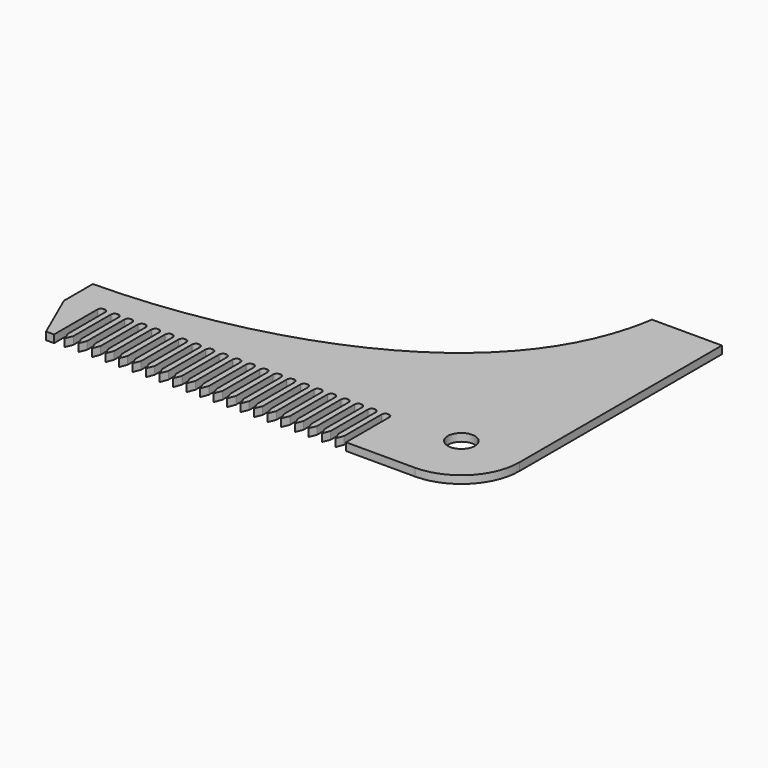
from build123d import *

# Parameters (mm, degrees)
F1_DEPTH = 2
F2_R     = 3.5
F3_DEPTH = 25


# Not quite as in the source:
# - a feature names something its author has since deleted; it is built from what else it names


with BuildPart() as f1:
    # F0 (on Top) → F1 (new body)
    with BuildSketch(Plane.XY):
        with BuildLine():
            ThreePointArc((-15.75, -19.0369902551), (-15.0428932188, -19.3298834739), (-14.75, -20.0369902551))
            Line((-14.75, -20.0369902551), (-14.75, -34))
            Line((-14.75, -34), (3.0843058825, -34))
            ThreePointArc((3.0843058825, -34), (13.6909076003, -29.6066017178), (18.0843058825, -19))
            Line((18.0843058825, -19), (18.0843058825, 46.4938916266))
            Line((18.0843058825, 46.4938916266), (0, 46.4938916266))
            add(Edge.make_bspline(
                [(-97.9156941175, -11.8882479146), (-60.4824349284, -11.5448236465), (-6.9082397968, 2.1921501029), (0, 46.4938916266)],
                knots=[0, 0, 0, 0, 113.9998130346, 113.9998130346, 113.9998130346, 113.9998130346], degree=3))
            Line((-97.9156941175, -11.8882479146), (-97.9156941175, -21.2501913908))
            Line((-97.9156941175, -21.2501913908), (-92.3223271966, -34))
            Line((-92.3223271966, -34), (-90.25, -34))
            Line((-90.25, -34), (-90.25, -32.1302767694))
            Line((-90.25, -32.1302767694), (-90.25, -20.0369902551))
            ThreePointArc((-90.25, -20.0369902551), (-89.9571067812, -19.3298834739), (-89.25, -19.0369902551))
            ThreePointArc((-89.25, -19.0369902551), (-88.5428932188, -19.3298834739), (-88.25, -20.0369902551))
            Line((-88.25, -20.0369902551), (-88.25, -32.1302767694))
            Line((-88.25, -32.1302767694), (-87.5, -34))
            Line((-87.5, -34), (-86.75, -32.1302767694))
            Line((-86.75, -32.1302767694), (-86.75, -20.0369902551))
            ThreePointArc((-86.75, -20.0369902551), (-86.4571067812, -19.3298834739), (-85.75, -19.0369902551))
            ThreePointArc((-85.75, -19.0369902551), (-85.0428932188, -19.3298834739), (-84.75, -20.0369902551))
            Line((-84.75, -20.0369902551), (-84.75, -32.1025866866))
            Line((-84.75, -32.1025866866), (-84, -34))
            Line((-84, -34), (-83.25, -32.1025866866))
            Line((-83.25, -32.1025866866), (-83.25, -20.0369902551))
            ThreePointArc((-83.25, -20.0369902551), (-82.9571067812, -19.3298834739), (-82.25, -19.0369902551))
            ThreePointArc((-82.25, -19.0369902551), (-81.5428932188, -19.3298834739), (-81.25, -20.0369902551))
            Line((-81.25, -20.0369902551), (-81.25, -32.0932865143))
            Line((-81.25, -32.0932865143), (-80.5, -34))
            Line((-80.5, -34), (-79.75, -32.0932865143))
            Line((-79.75, -32.0932865143), (-79.75, -20.0369902551))
            ThreePointArc((-79.75, -20.0369902551), (-79.4571067812, -19.3298834739), (-78.75, -19.0369902551))
            ThreePointArc((-78.75, -19.0369902551), (-78.0428932188, -19.3298834739), (-77.75, -20.0369902551))
            Line((-77.75, -20.0369902551), (-77.75, -32.0655964315))
            Line((-77.75, -32.0655964315), (-77, -34))
            Line((-77, -34), (-76.25, -32.0655964315))
            Line((-76.25, -32.0655964315), (-76.25, -20.0369902551))
            ThreePointArc((-76.25, -20.0369902551), (-75.9571067812, -19.3298834739), (-75.25, -19.0369902551))
            ThreePointArc((-75.25, -19.0369902551), (-74.5428932188, -19.3298834739), (-74.25, -20.0369902551))
            Line((-74.25, -20.0369902551), (-74.25, -32.0655964315))
            Line((-74.25, -32.0655964315), (-73.5, -34))
            Line((-73.5, -34), (-72.75, -32.0655964315))
            Line((-72.75, -32.0655964315), (-72.75, -20.0369902551))
            ThreePointArc((-72.75, -20.0369902551), (-72.4571067812, -19.3298834739), (-71.75, -19.0369902551))
            ThreePointArc((-71.75, -19.0369902551), (-71.0428932188, -19.3298834739), (-70.75, -20.0369902551))
            Line((-70.75, -20.0369902551), (-70.75, -32.0932865143))
            Line((-70.75, -32.0932865143), (-70, -34))
            Line((-70, -34), (-69.25, -32.0932865143))
            Line((-69.25, -32.0932865143), (-69.25, -20.0369902551))
            ThreePointArc((-69.25, -20.0369902551), (-68.9571067812, -19.3298834739), (-68.25, -19.0369902551))
            ThreePointArc((-68.25, -19.0369902551), (-67.5428932188, -19.3298834739), (-67.25, -20.0369902551))
            Line((-67.25, -20.0369902551), (-67.25, -32.0932865143))
            Line((-67.25, -32.0932865143), (-66.5, -34))
            Line((-66.5, -34), (-65.75, -32.0932865143))
            Line((-65.75, -32.0932865143), (-65.75, -20.0369902551))
            ThreePointArc((-65.75, -20.0369902551), (-65.4571067812, -19.3298834739), (-64.75, -19.0369902551))
            ThreePointArc((-64.75, -19.0369902551), (-64.0428932188, -19.3298834739), (-63.75, -20.0369902551))
            Line((-63.75, -20.0369902551), (-63.75, -32.0655964315))
            Line((-63.75, -32.0655964315), (-63, -34))
            Line((-63, -34), (-62.25, -32.0655964315))
            Line((-62.25, -32.0655964315), (-62.25, -20.0369902551))
            ThreePointArc((-62.25, -20.0369902551), (-61.9571067812, -19.3298834739), (-61.25, -19.0369902551))
            ThreePointArc((-61.25, -19.0369902551), (-60.5428932188, -19.3298834739), (-60.25, -20.0369902551))
            Line((-60.25, -20.0369902551), (-60.25, -32.0655964315))
            Line((-60.25, -32.0655964315), (-59.5, -34))
            Line((-59.5, -34), (-58.75, -32.0655964315))
            Line((-58.75, -32.0655964315), (-58.75, -20.0369902551))
            ThreePointArc((-58.75, -20.0369902551), (-58.4571067812, -19.3298834739), (-57.75, -19.0369902551))
            ThreePointArc((-57.75, -19.0369902551), (-57.0428932188, -19.3298834739), (-56.75, -20.0369902551))
            Line((-56.75, -20.0369902551), (-56.75, -32.0932865143))
            Line((-56.75, -32.0932865143), (-56, -34))
            Line((-56, -34), (-55.25, -32.0932865143))
            Line((-55.25, -32.0932865143), (-55.25, -20.0369902551))
            ThreePointArc((-55.25, -20.0369902551), (-54.9571067812, -19.3298834739), (-54.25, -19.0369902551))
            ThreePointArc((-54.25, -19.0369902551), (-53.5428932188, -19.3298834739), (-53.25, -20.0369902551))
            Line((-53.25, -20.0369902551), (-53.25, -32.0932865143))
            Line((-53.25, -32.0932865143), (-52.5, -34))
            Line((-52.5, -34), (-51.75, -32.0932865143))
            Line((-51.75, -32.0932865143), (-51.75, -20.0369902551))
            ThreePointArc((-51.75, -20.0369902551), (-51.4571067812, -19.3298834739), (-50.75, -19.0369902551))
            ThreePointArc((-50.75, -19.0369902551), (-50.0428932188, -19.3298834739), (-49.75, -20.0369902551))
            Line((-49.75, -20.0369902551), (-49.75, -32.0655964315))
            Line((-49.75, -32.0655964315), (-49, -34))
            Line((-49, -34), (-48.25, -32.0655964315))
            Line((-48.25, -32.0655964315), (-48.25, -20.0369902551))
            ThreePointArc((-48.25, -20.0369902551), (-47.9571067812, -19.3298834739), (-47.25, -19.0369902551))
            ThreePointArc((-47.25, -19.0369902551), (-46.5428932188, -19.3298834739), (-46.25, -20.0369902551))
            Line((-46.25, -20.0369902551), (-46.25, -32.0655964315))
            Line((-46.25, -32.0655964315), (-45.5, -34))
            Line((-45.5, -34), (-44.75, -32.0655964315))
            Line((-44.75, -32.0655964315), (-44.75, -20.0369902551))
            ThreePointArc((-44.75, -20.0369902551), (-44.4571067812, -19.3298834739), (-43.75, -19.0369902551))
            ThreePointArc((-43.75, -19.0369902551), (-43.0428932188, -19.3298834739), (-42.75, -20.0369902551))
            Line((-42.75, -20.0369902551), (-42.75, -32.176785171))
            Line((-42.75, -32.176785171), (-42, -34))
            Line((-42, -34), (-41.25, -32.176785171))
            Line((-41.25, -32.176785171), (-41.25, -20.0369902551))
            ThreePointArc((-41.25, -20.0369902551), (-40.9571067812, -19.3298834739), (-40.25, -19.0369902551))
            ThreePointArc((-40.25, -19.0369902551), (-39.5428932188, -19.3298834739), (-39.25, -20.0369902551))
            Line((-39.25, -20.0369902551), (-39.25, -32.176785171))
            Line((-39.25, -32.176785171), (-38.5, -34))
            Line((-38.5, -34), (-37.75, -32.176785171))
            Line((-37.75, -32.176785171), (-37.75, -20.0369902551))
            ThreePointArc((-37.75, -20.0369902551), (-37.4571067812, -19.3298834739), (-36.75, -19.0369902551))
            ThreePointArc((-36.75, -19.0369902551), (-36.0428932188, -19.3298834739), (-35.75, -20.0369902551))
            Line((-35.75, -20.0369902551), (-35.75, -32.1490950882))
            Line((-35.75, -32.1490950882), (-35, -34))
            Line((-35, -34), (-34.25, -32.1490950882))
            Line((-34.25, -32.1490950882), (-34.25, -20.0369902551))
            ThreePointArc((-34.25, -20.0369902551), (-33.9571067812, -19.3298834739), (-33.25, -19.0369902551))
            ThreePointArc((-33.25, -19.0369902551), (-32.5428932188, -19.3298834739), (-32.25, -20.0369902551))
            Line((-32.25, -20.0369902551), (-32.25, -32.1490950882))
            Line((-32.25, -32.1490950882), (-31.5, -34))
            Line((-31.5, -34), (-30.75, -32.1490950882))
            Line((-30.75, -32.1490950882), (-30.75, -20.0369902551))
            ThreePointArc((-30.75, -20.0369902551), (-30.4571067812, -19.3298834739), (-29.75, -19.0369902551))
            ThreePointArc((-29.75, -19.0369902551), (-29.0428932188, -19.3298834739), (-28.75, -20.0369902551))
            Line((-28.75, -20.0369902551), (-28.75, -32.1209765971))
            Line((-28.75, -32.1209765971), (-28, -34))
            Line((-28, -34), (-27.25, -32.1209765971))
            Line((-27.25, -32.1209765971), (-27.25, -20.0369902551))
            ThreePointArc((-27.25, -20.0369902551), (-26.9571067812, -19.3298834739), (-26.25, -19.0369902551))
            ThreePointArc((-26.25, -19.0369902551), (-25.5428932188, -19.3298834739), (-25.25, -20.0369902551))
            Line((-25.25, -20.0369902551), (-25.25, -32.1209765971))
            Line((-25.25, -32.1209765971), (-24.5, -34))
            Line((-24.5, -34), (-23.75, -32.1209765971))
            Line((-23.75, -32.1209765971), (-23.75, -20.0369902551))
            ThreePointArc((-23.75, -20.0369902551), (-23.4571067812, -19.3298834739), (-22.75, -19.0369902551))
            ThreePointArc((-22.75, -19.0369902551), (-22.0428932188, -19.3298834739), (-21.75, -20.0369902551))
            Line((-21.75, -20.0369902551), (-21.75, -32.0932865143))
            Line((-21.75, -32.0932865143), (-21, -34))
            Line((-21, -34), (-20.25, -32.0932865143))
            Line((-20.25, -32.0932865143), (-20.25, -20.0369902551))
            ThreePointArc((-20.25, -20.0369902551), (-19.9571067812, -19.3298834739), (-19.25, -19.0369902551))
            ThreePointArc((-19.25, -19.0369902551), (-18.5428932188, -19.3298834739), (-18.25, -20.0369902551))
            Line((-18.25, -20.0369902551), (-18.25, -32.0932865143))
            Line((-18.25, -32.0932865143), (-17.5, -34))
            Line((-17.5, -34), (-16.75, -32.0932865143))
            Line((-16.75, -32.0932865143), (-16.75, -20.0369902551))
            ThreePointArc((-16.75, -20.0369902551), (-16.4571067812, -19.3298834739), (-15.75, -19.0369902551))
        make_face()
    extrude(amount=F1_DEPTH)

    # F2 (on face) → F3 (cut)
    with BuildSketch(Plane.XY.offset(2)):
        with Locations((3.0843058825, -19)):
            Circle(F2_R)
    extrude(amount=-F3_DEPTH, mode=Mode.SUBTRACT)


solid = f1.part
